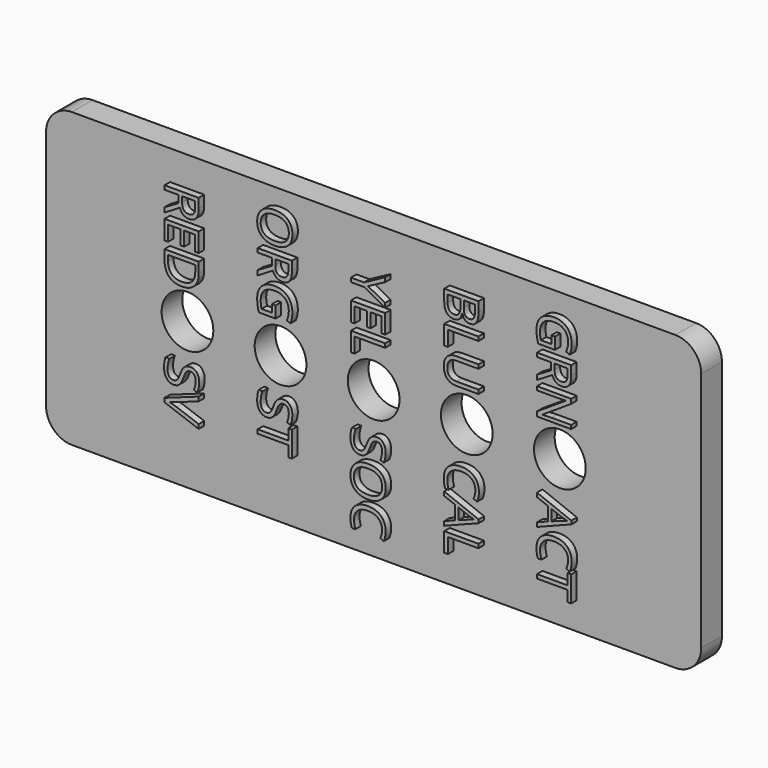
from build123d import *

# Parameters (mm, degrees)
F0_R         = 1.5
F1_DEPTH     = 1.5
F2_TEXT_SIZE = 2.7777777778
F3_DEPTH     = 0.4


# Not quite as in the source:
# - Text() gives the source's letters only with a copy of the font that has no kerning and outlines rounded to 1/6400 em; it was checked with that copy


with BuildPart() as f1:
    # F0 (on Front) → F1 (new body)
    with BuildSketch(Plane.XZ):
        with BuildLine():
            Line((-53.7273784454, 33.8626480699), (-88.7273784454, 33.8626480699))
            ThreePointArc((-88.7273784454, 33.8626480699), (-89.7880386171, 33.4233082416), (-90.2273784454, 32.3626480699))
            Line((-90.2273784454, 32.3626480699), (-90.2273784454, 18.3626480699))
            ThreePointArc((-90.2273784454, 18.3626480699), (-89.7880386171, 17.3019878981), (-88.7273784454, 16.8626480699))
            Line((-88.7273784454, 16.8626480699), (-53.7273784454, 16.8626480699))
            ThreePointArc((-53.7273784454, 16.8626480699), (-52.6667182736, 17.3019878981), (-52.2273784454, 18.3626480699))
            Line((-52.2273784454, 18.3626480699), (-52.2273784454, 32.3626480699))
            ThreePointArc((-52.2273784454, 32.3626480699), (-52.6667182736, 33.4233082416), (-53.7273784454, 33.8626480699))
        make_face()
        with Locations((-82.0273784454, 25.3626480699)):
            Circle(F0_R, mode=Mode.SUBTRACT)
        with Locations((-76.6273784454, 25.369741105)):
            Circle(F0_R, mode=Mode.SUBTRACT)
        with Locations((-71.2273784454, 25.3626480699)):
            Circle(F0_R, mode=Mode.SUBTRACT)
        with Locations((-65.8273784454, 25.3626480699)):
            Circle(F0_R, mode=Mode.SUBTRACT)
        with Locations((-60.4273784454, 25.3626480699)):
            Circle(F0_R, mode=Mode.SUBTRACT)
    extrude(amount=F1_DEPTH)

    # F2 (on face) → F3 (join)
    with BuildSketch(Plane.XZ.offset(1.5)):
        with Locations(Location((-61.4341739151, 32.9148996916), (0, 0, -90))):
            Text('GRN     ACT', F2_TEXT_SIZE, font='Open Sans', text_align=(TextAlign.LEFT, TextAlign.BOTTOM))
        with Locations(Location((-66.8128218113, 32.4086834685), (0, 0, -90))):
            Text('BLU     CAL', F2_TEXT_SIZE, font='Open Sans', text_align=(TextAlign.LEFT, TextAlign.BOTTOM))
        with Locations(Location((-72.2243047515, 31.6009602989), (0, 0, -90))):
            Text('YEL     SOC', F2_TEXT_SIZE, font='Open Sans', text_align=(TextAlign.LEFT, TextAlign.BOTTOM))
        with Locations(Location((-77.6357828508, 33.1233694025), (0, 0, -90))):
            Text('ORG     ST', F2_TEXT_SIZE, font='Open Sans', text_align=(TextAlign.LEFT, TextAlign.BOTTOM))
        with Locations(Location((-83.0374098945, 32.4123264269), (0, 0, -90))):
            Text('RED     SV', F2_TEXT_SIZE, font='Open Sans', text_align=(TextAlign.LEFT, TextAlign.BOTTOM))
    extrude(amount=F3_DEPTH)


solid = f1.part
